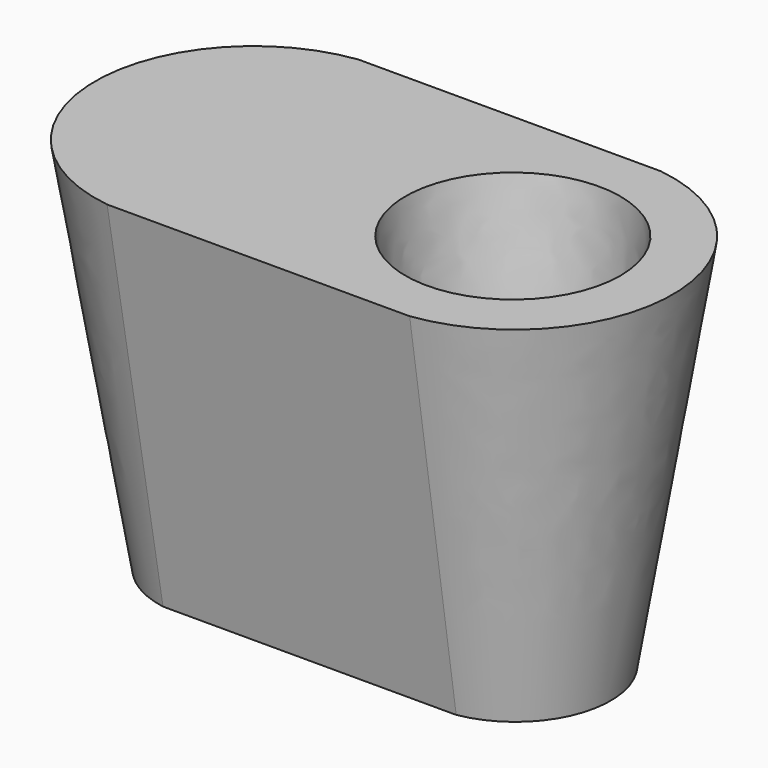
from build123d import *

# Parameters (mm, degrees)
F4_R = 21.6754644631
F5_R = 13.3144971064


with BuildPart() as f3:
    # F2 (on face) → F3 section 0
    with BuildSketch(Plane.XY.offset(76.2)):
        with BuildLine():
            Line((20.7843769666, 44.2757006465), (-40.2313820243, 44.2757006465))
            ThreePointArc((-40.2313820243, 44.2757006465), (-67.9658874869, 12.6128514133), (-40.2313820243, -19.0499978198))
            Line((-40.2313820243, -19.0499978198), (20.7843769666, -19.0499978198))
            ThreePointArc((20.7843769666, -19.0499978198), (48.5188824293, 12.6128514133), (20.7843769666, 44.2757006465))
        make_face()
    # F0 (on Top) → F3 section 1
    with BuildSketch(Plane.XY):
        with BuildLine():
            ThreePointArc((-39.1175734429, 31.5757045358), (-55.0984784521, 12.6128522679), (-39.1175734429, -6.35))
            Line((-39.1175734429, -6.35), (20.0053925244, -6.35))
            ThreePointArc((20.0053925244, -6.35), (35.9862975337, 12.6128522679), (20.0053925244, 31.5757045358))
            Line((20.0053925244, 31.5757045358), (-39.1175734429, 31.5757045358))
        make_face()
    loft()

    # F4 (on face) → F6 section 0
    with BuildSketch(Plane.XY.offset(76.2)):
        with Locations((16.3852963597, 12.4639989808)):
            Circle(F4_R)
    # F5 (on Top) → F6 section 1
    with BuildSketch(Plane.XY):
        with Locations((16.5599323809, 12.6425297931)):
            Circle(F5_R)
    loft(mode=Mode.SUBTRACT)


solid = f3.part
